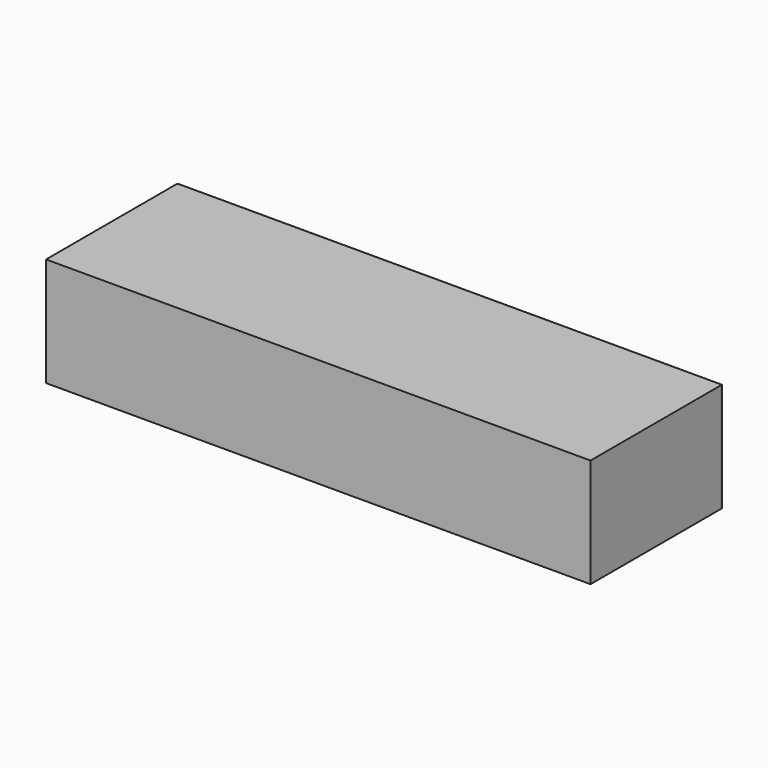
from build123d import *

# Parameters (mm, degrees)
F0_W     = 1524
F0_H     = 304.8
F1_DEPTH = 457.2
F2_T     = -2.54
F4_W     = 760.2678739185
F4_H     = 304.7950782727
F5_DEPTH = 2.54
F6_R     = 24.9213487402
F7_DEPTH = 2.54
F8_W     = 762.243449688
F8_H     = 304.7996152788
F9_DEPTH = 2.54


with BuildPart() as f1:
    # F0 (on Front) → F1 (new body)
    with BuildSketch(Plane.XZ):
        with Locations((725.2281959057, 152.4)):
            Rectangle(F0_W, F0_H)
    extrude(amount=F1_DEPTH)

    # F2
    f2_openings = [f1.faces().sort_by_distance(p)[0] for p in [
        (725.228196, 0, 152.4),
    ]]
    offset(amount=F2_T, openings=f2_openings)


with BuildPart() as f5:
    # F4 (on offset) → F5 (new body)
    with BuildSketch(Plane.XZ.offset(-2.54)):
        with Locations((344.8506124159, 152.3975391363)):
            Rectangle(F4_W, F4_H)
    extrude(amount=F5_DEPTH)

    # F6 (on offset) → F7, piece 2 (join)
    with BuildSketch(Plane.XZ.offset(-2.54)):
        with Locations((643.3112621307, 152.4)):
            Circle(F6_R)
    extrude(amount=-F7_DEPTH)


with BuildPart() as f7:
    # F6 (on offset) → F7 (new body)
    with BuildSketch(Plane.XZ.offset(-2.54)):
        with Locations((806.498169899, 152.4)):
            Circle(F6_R)
    extrude(amount=-F7_DEPTH)


with BuildPart() as f9:
    # F8 (on offset) → F9 (new body)
    with BuildSketch(Plane.XZ.offset(-2.54)):
        with Locations((1106.1064302921, 152.3997788951)):
            Rectangle(F8_W, F8_H)
    extrude(amount=F9_DEPTH)


solid = Compound([f1.part, f5.part, f7.part, f9.part])
